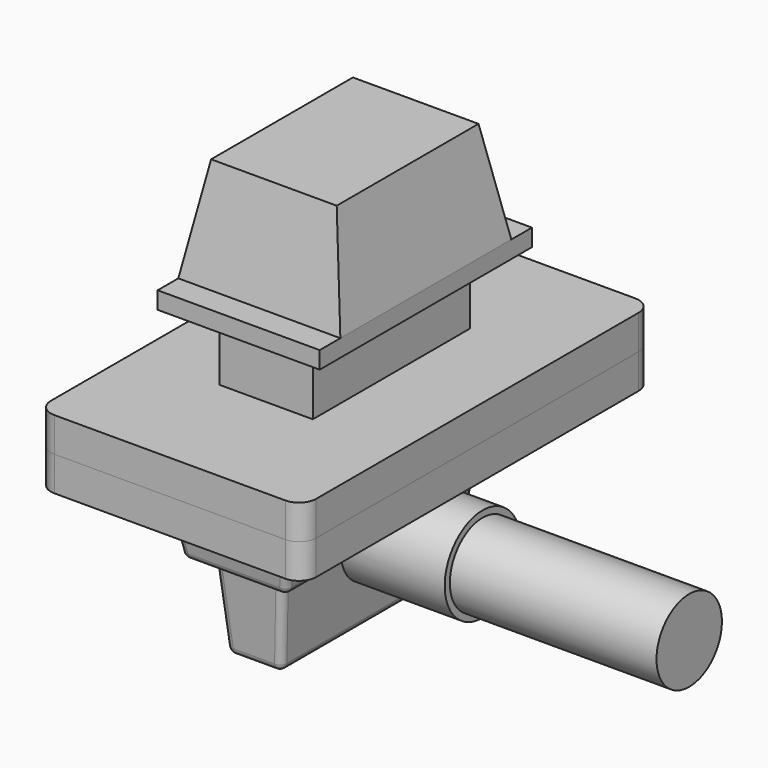
from build123d import *

# Parameters (mm, degrees)
F0_W           = 76.2
F0_H           = 203.2
F1_DEPTH       = 50.8
F1_TAPER       = -10
F2_W           = 195.71482124
F2_H           = 322.71482124
F2_W_2         = 94.11482124
F2_H_2         = 221.11482124
F3_DEPTH       = 25.4
F4_DEPTH       = 25.4
F5_R           = 12.7
F5_2_R         = 12.7
F6_W           = 50.7999997139
F6_H           = 177.7999997139
F7_DEPTH       = 63.5
F7_TAPER       = 5
F8_R           = 5.08
F9_W           = 68.71482124
F9_H           = 144.91482124
F10_DEPTH      = 50.8
F11_W          = 119.51482124
F11_H          = 195.71482124
F11_W_2        = 68.71482124
F11_H_2        = 144.91482124
F12_DEPTH      = 12.7
F13_W          = 119.51482124
F13_H          = 157.61482124
F14_DEPTH      = 76.2
F14_TAPER      = 10
F15_R          = 34.925
F16_DEPTH      = 101.6
F16_DEPTH_BACK = 101.6
F17_R          = 30.1625
F18_DEPTH      = 152.4


with BuildPart() as f1:
    # F0 (on Top) → F1 (new body)
    with BuildSketch(Plane.XY):
        Rectangle(F0_W, F0_H)
    extrude(amount=F1_DEPTH, taper=F1_TAPER)

    # F2 (on face) → F3 (join)
    with BuildSketch(Plane.XY.offset(50.8)):
        Rectangle(F2_W, F2_H)
        Rectangle(F2_W_2, F2_H_2, mode=Mode.SUBTRACT)
        Rectangle(F2_W_2, F2_H_2)
    extrude(amount=F3_DEPTH)


with BuildPart() as f4:
    # F4 (new): a face of the model
    f4_faces = [f1.part.faces().sort_by_distance(p)[0] for p in [
        (0, 0, 76.2),
    ]]
    extrude(f4_faces, amount=F4_DEPTH)

    # F5#2
    f5_2_edges = [f4.edges().sort_by_distance(p)[0] for p in [
        (-97.857411, -161.357411, 88.9),
        (97.857411, -161.357411, 88.9),
        (97.857411, 161.357411, 88.9),
        (-97.857411, 161.357411, 88.9),
    ]]
    fillet(f5_2_edges, radius=F5_2_R)

    # F9 (on face) → F10 (join)
    with BuildSketch(Plane.XY.offset(101.6)):
        Rectangle(F9_W, F9_H)
    extrude(amount=F10_DEPTH)

    # F11 (on face) → F12 (join)
    with BuildSketch(Plane.XY.offset(152.4)):
        Rectangle(F11_W, F11_H)
        Rectangle(F11_W_2, F11_H_2, mode=Mode.SUBTRACT)
        Rectangle(F11_W_2, F11_H_2)
    extrude(amount=F12_DEPTH)

    # F13 (on face) → F14 (join)
    with BuildSketch(Plane.XY.offset(165.1)):
        Rectangle(F13_W, F13_H)
    extrude(amount=F14_DEPTH, taper=F14_TAPER)


with BuildPart() as f1_1:
    add(f1.part)

    # F5
    f5_edges = [f1_1.edges().sort_by_distance(p)[0] for p in [
        (97.857411, -161.357411, 63.5),
        (-97.857411, -161.357411, 63.5),
        (97.857411, 161.357411, 63.5),
        (-97.857411, 161.357411, 63.5),
    ]]
    fillet(f5_edges, radius=F5_R)

    # F6 (on face) → F7 (join)
    with BuildSketch(Plane(origin=(0, 0, 0), x_dir=(1, 0, 0), z_dir=(0, 0, -1))):
        Rectangle(F6_W, F6_H)
    extrude(amount=F7_DEPTH, taper=F7_TAPER)

    # F8
    f8_edges = [f1_1.edges().sort_by_distance(p)[0] for p in [
        (38.1, 0, 0),
        (19.84447, 0, -63.5),
        (22.622235, -86.122235, -31.75),
        (22.622235, 86.122235, -31.75),
        (42.578705, 106.078705, 25.4),
        (42.578705, -106.078705, 25.4),
        (0, -101.6, 0),
        (-42.578705, -106.078705, 25.4),
        (-22.622235, -86.122235, -31.75),
        (0, -83.34447, -63.5),
        (-19.84447, 0, -63.5),
        (-22.622235, 86.122235, -31.75),
        (-38.1, 0, 0),
        (-47.057411, 0, 50.8),
        (-42.578705, 106.078705, 25.4),
        (0, -110.557411, 50.8),
        (47.057411, 0, 50.8),
        (0, 110.557411, 50.8),
    ]]
    fillet(f8_edges, radius=F8_R)

    # F15 (on Right) → F16 (join, two sides)
    with BuildSketch(Plane.YZ) as f16_sk:
        Circle(F15_R)
    extrude(amount=F16_DEPTH)
    extrude(f16_sk.sketch, amount=-F16_DEPTH_BACK)

    # F17 (on face) → F18 (join)
    with BuildSketch(Plane.YZ.offset(101.6)):
        Circle(F17_R)
    extrude(amount=F18_DEPTH)


solid = Compound([f4.part, f1_1.part])
